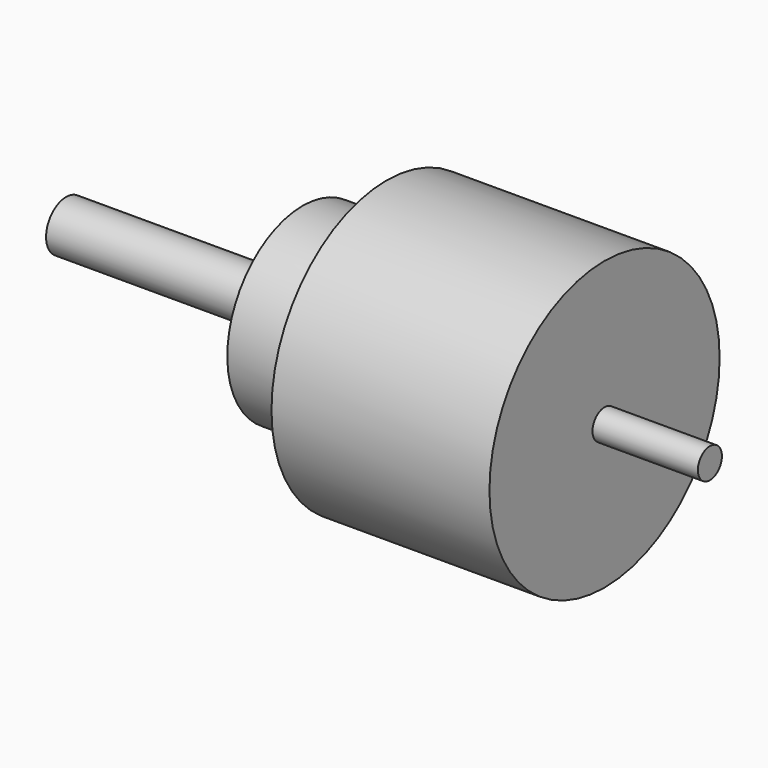
from build123d import *

# Parameters (mm, degrees)
F1_W = 10.51
F1_H = 1.5
F2_W = 38.31
F2_H = 1.5
F3_W = 23.6
F3_H = 2.5


with BuildPart() as f4:
    # F1 (on Front) → F4 (revolve)
    with BuildSketch(Plane.XZ):
        with Locations((5.255, 0.75)):
            Rectangle(F1_W, F1_H)
    revolve(axis=Axis((-21.6, 0, 0), (-1, 0, 0)))

    # F2 (on Front) → F5 (revolve)
    with BuildSketch(Plane.XZ):
        with Locations((-8.645, 0.75)):
            Rectangle(F2_W, F2_H)
    revolve(axis=Axis((-21.6, 0, 0), (-1, 0, 0)))


with BuildPart() as f4b:
    # F1 (on Front) → F4, piece 2 (revolve)
    with BuildSketch(Plane.XZ):
        Polygon((0, 14.35), (-21.7421161675, 14.35), (-24.6, 9.4), (-24.6, 1.5), (0, 1.5), align=None)
    revolve(axis=Axis((-21.6, 0, 0), (-1, 0, 0)))


with BuildPart() as f6:
    # F3 (on Front) → F6 (revolve)
    with BuildSketch(Plane.XZ):
        with Locations((-41.91, 1.25)):
            Rectangle(F3_W, F3_H)
        Polygon((-24.6, 9.4), (-30.11, 9.4), (-30.11, 2.5), (-30.11, 0), (-24.6, 0), align=None)
    revolve(axis=Axis((-21.6, 0, 0), (-1, 0, 0)))


solid = Compound([f4.part, f4b.part, f6.part])
